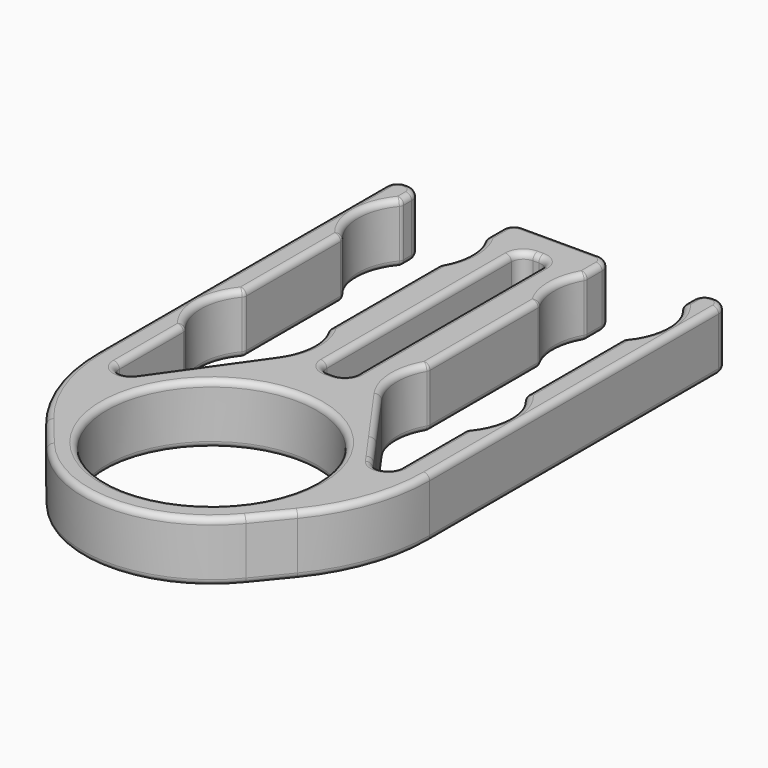
from build123d import *

# Parameters (mm, degrees)
F0_R         = 8.75
F0_W         = 2.5
F0_H         = 21.2536069062
F1_DEPTH     = 5
F2_R         = 1
F3_R         = 0.49999
F4_T1_DEPTH  = 5
F4_T4_ANGLE  = 39.3414951805
F4_T6_ANGLE  = 39.3414951805
F4_T8_ANGLE  = 39.3414951805
F4_T10_ANGLE = 39.3414951805


# Not quite as in the source:
# - a fillet or chamfer that OpenCascade refuses, or shapes differently, is made with other operations: its cross-section is extruded or revolved along the edge and cut away or added
# - a fillet or chamfer is up to 0.001 mm smaller than in the source, because OpenCascade refuses the exact size


with BuildPart() as f1:
    # F0 (on Top) → F1 (new body)
    with BuildSketch(Plane.XY):
        with BuildLine():
            ThreePointArc((-3.525, -3.1087577905), (-4.7, 0), (-3.525, 3.1087577905))
            Line((-3.525, 3.1087577905), (-3.525, 13.2912422095))
            ThreePointArc((-3.525, 13.2912422095), (-4.7, 16.4), (-3.525, 19.5087577905))
            Line((-3.525, 19.5087577905), (-3.525, 21.5087577905))
            Line((-3.525, 21.5087577905), (-5.7, 21.5087577905))
            Line((-5.7, 21.5087577905), (-5.7, 0))
            Line((-5.7, 0), (-5.7, -15))
            Line((-5.7, -15), (-0.1138489209, -21.8148672857))
            ThreePointArc((-0.1138489209, -21.8148672857), (8.2, -25.75), (16.5138489209, -21.8148672857))
            Line((16.5138489209, -21.8148672857), (22.1, -15))
            Line((22.1, -15), (22.1, 0))
            Line((22.1, 0), (22.1, 21.5087577905))
            Line((22.1, 21.5087577905), (19.925, 21.5087577905))
            Line((19.925, 21.5087577905), (19.925, 19.5087577905))
            ThreePointArc((19.925, 19.5087577905), (21.1, 16.4), (19.925, 13.2912422095))
            Line((19.925, 13.2912422095), (19.925, 3.1087577905))
            ThreePointArc((19.925, 3.1087577905), (21.1, 0), (19.925, -3.1087577905))
            Line((19.925, -3.1087577905), (19.925, -13.1087577905))
            Line((19.925, -13.1087577905), (17.6966700997, -9.9625644404))
            Line((17.6966700997, -9.9625644404), (16.1036863409, -7.713420403))
            Line((16.1036863409, -7.713420403), (12.5645563007, -2.7164998857))
            ThreePointArc((12.5645563007, -2.7164998857), (11.703188731, -0.1731008479), (12.375, 2.4268034531))
            Line((12.375, 2.4268034531), (12.375, 13.9731965469))
            ThreePointArc((12.375, 13.9731965469), (11.7, 16.4), (12.375, 18.8268034531))
            Line((12.375, 18.8268034531), (12.375, 21.5087577905))
            Line((12.375, 21.5087577905), (8.2, 21.5087577905))
            Line((8.2, 21.5087577905), (4.025, 21.5087577905))
            Line((4.025, 21.5087577905), (4.025, 18.8268034531))
            ThreePointArc((4.025, 18.8268034531), (4.7, 16.4), (4.025, 13.9731965469))
            Line((4.025, 13.9731965469), (4.025, 2.4268034531))
            ThreePointArc((4.025, 2.4268034531), (4.696811269, -0.1731008479), (3.8354436993, -2.7164998857))
            Line((3.8354436993, -2.7164998857), (0.2963136591, -7.713420403))
            Line((0.2963136591, -7.713420403), (-1.2966700997, -9.9625644404))
            Line((-1.2966700997, -9.9625644404), (-3.525, -13.1087577905))
            Line((-3.525, -13.1087577905), (-3.525, -3.1087577905))
        make_face()
        with Locations((8.2, -15)):
            Circle(F0_R, mode=Mode.SUBTRACT)
        with Locations((8.2, 8.2)):
            Rectangle(F0_W, F0_H, mode=Mode.SUBTRACT)
    extrude(amount=F1_DEPTH)

    # F2
    f2_edges = [f1.edges().sort_by_distance(p)[0] for p in [
        (-3.525, -13.108758, 2.5),
        (19.925, -13.108758, 2.5),
        (4.025, 21.508758, 2.5),
        (-5.7, 21.508758, 2.5),
        (-3.525, 21.508758, 2.5),
        (12.375, 21.508758, 2.5),
        (19.925, 21.508758, 2.5),
        (22.1, 21.508758, 2.5),
        (6.95, -2.426803, 2.5),
        (9.45, -2.426803, 2.5),
        (9.45, 18.826803, 2.5),
        (6.95, 18.826803, 2.5),
    ]]
    fillet(f2_edges, radius=F2_R)

    # F3 (radius 0.5 in the source; OpenCascade refuses exactly that, so slightly less here)
    f3_edges = [f1.edges().sort_by_distance(p)[0] for p in [
        (4.025, 19.667781, 5),
        (4.317893, 21.215865, 5),
        (4.7, 16.4, 5),
        (8.2, 21.508758, 5),
        (4.025, 8.2, 5),
        (12.082107, 21.215865, 5),
        (4.696811, -0.173101, 5),
        (12.375, 19.667781, 5),
        (1.063248, -6.630581, 5),
        (11.7, 16.4, 5),
        (-2.828272, -10.919588, 5),
        (12.375, 8.2, 5),
        (-3.525, -6.537721, 5),
        (11.703189, -0.173101, 5),
        (-4.7, 0, 5),
        (15.336752, -6.630581, 5),
        (-3.525, 8.2, 5),
        (19.228272, -10.919588, 5),
        (-4.7, 16.4, 5),
        (19.925, -6.537721, 5),
        (-3.525, 20.008758, 5),
        (21.1, 0, 5),
        (-3.817893, 21.215865, 5),
        (19.925, 8.2, 5),
        (-4.6125, 21.508758, 5),
        (21.1, 16.4, 5),
        (-5.407107, 21.215865, 5),
        (19.925, 20.008758, 5),
        (-5.7, 2.754379, 5),
        (20.217893, 21.215865, 5),
        (-2.906924, -18.407434, 5),
        (21.0125, 21.508758, 5),
        (8.2, -25.75, 5),
        (21.807107, 21.215865, 5),
        (19.306924, -18.407434, 5),
        (22.1, 2.754379, 5),
        (-0.55, -15, 5),
        (8.2, 18.826803, 5),
        (7.242893, 18.53391, 5),
        (9.157107, 18.53391, 5),
        (6.95, 8.2, 5),
        (9.45, 8.2, 5),
        (7.242893, -2.13391, 5),
        (9.157107, -2.13391, 5),
        (8.2, -2.426803, 5),
        (4.025, 19.667781, 0),
        (4.317893, 21.215865, 0),
        (4.7, 16.4, 0),
        (8.2, 21.508758, 0),
        (4.025, 8.2, 0),
        (12.082107, 21.215865, 0),
        (4.696811, -0.173101, 0),
        (12.375, 19.667781, 0),
        (1.063248, -6.630581, 0),
        (11.7, 16.4, 0),
        (-2.828272, -10.919588, 0),
        (12.375, 8.2, 0),
        (-3.525, -6.537721, 0),
        (11.703189, -0.173101, 0),
        (-4.7, 0, 0),
        (15.336752, -6.630581, 0),
        (-3.525, 8.2, 0),
        (19.228272, -10.919588, 0),
        (-4.7, 16.4, 0),
        (19.925, -6.537721, 0),
        (-3.525, 20.008758, 0),
        (21.1, 0, 0),
        (-3.817893, 21.215865, 0),
        (19.925, 8.2, 0),
        (-4.6125, 21.508758, 0),
        (21.1, 16.4, 0),
        (-5.407107, 21.215865, 0),
        (19.925, 20.008758, 0),
        (-5.7, 2.754379, 0),
        (20.217893, 21.215865, 0),
        (-2.906924, -18.407434, 0),
        (21.0125, 21.508758, 0),
        (8.2, -25.75, 0),
        (21.807107, 21.215865, 0),
        (19.306924, -18.407434, 0),
        (22.1, 2.754379, 0),
        (-0.55, -15, 0),
        (8.2, 18.826803, 0),
        (7.242893, 18.53391, 0),
        (9.157107, 18.53391, 0),
        (6.95, 8.2, 0),
        (9.45, 8.2, 0),
        (7.242893, -2.13391, 0),
        (9.157107, -2.13391, 0),
        (8.2, -2.426803, 0),
        (-3.525, 3.108758, 2.5),
        (-3.525, -3.108758, 2.5),
        (-3.525, 13.291242, 2.5),
        (-3.525, 19.508758, 2.5),
        (12.375, 13.973197, 2.5),
        (12.375, 18.826803, 2.5),
        (12.375, 2.426803, 2.5),
        (4.025, 2.426803, 2.5),
        (4.025, 13.973197, 2.5),
        (4.025, 18.826803, 2.5),
        (19.925, 19.508758, 2.5),
        (19.925, 13.291242, 2.5),
        (19.925, -3.108758, 2.5),
        (19.925, 3.108758, 2.5),
    ]]
    fillet(f3_edges, radius=F3_R)

    # F4: fillet of radius 15 on 2 edges, made by hand

    # F4_s2 → F4_t1 (cut)
    with BuildSketch(Plane.XY):
        with BuildLine():
            ThreePointArc((22.1, -9.6378609215), (21.2246378957, -14.6870791102), (18.7007194245, -19.1469780643))
            Line((18.7007194245, -19.1469780643), (22.1, -15))
            Line((22.1, -15), (22.1, -9.6378609215))
        make_face()
        with BuildLine():
            ThreePointArc((-2.3007194245, -19.1469780643), (-4.8246378957, -14.6870791102), (-5.7, -9.6378609215))
            Line((-5.7, -9.6378609215), (-5.7, -15))
            Line((-5.7, -15), (-2.3007194245, -19.1469780643))
        make_face()
    extrude(amount=F4_T1_DEPTH, mode=Mode.SUBTRACT)

    # F4_s3 → F4_t4 (revolve, cut)
    with BuildSketch(Plane(origin=(8.4627300816, -10.32417161, 0), x_dir=(0, 0, 1), z_dir=(0.6339411429, -0.773381295, 0))):
        with BuildLine():
            ThreePointArc((0, 13.4174005241), (0.1464436805, 13.7709468436), (0.49999, 13.9173905241))
            Line((0.49999, 13.9173905241), (0, 13.9173905241))
            Line((0, 13.9173905241), (0, 13.4174005241))
        make_face()
    revolve(axis=Axis((9.3, -9.6378609215, 0), (0, 0, -1)), revolution_arc=F4_T4_ANGLE, mode=Mode.SUBTRACT)

    # F4_s5 → F4_t6 (revolve, cut)
    with BuildSketch(Plane.XZ.offset(9.6378609215)):
        with BuildLine():
            ThreePointArc((-5.20001, 5), (-5.5535563195, 4.8535563195), (-5.7, 4.50001))
            Line((-5.7, 4.50001), (-5.7, 5))
            Line((-5.7, 5), (-5.20001, 5))
        make_face()
    revolve(axis=Axis((9.3, -9.6378609215, 5), (0, 0, 1)), revolution_arc=F4_T6_ANGLE, mode=Mode.SUBTRACT)

    # F4_s7 → F4_t8 (revolve, cut)
    with BuildSketch(Plane.XZ.offset(9.6378609215)):
        with BuildLine():
            ThreePointArc((21.60001, 0), (21.9535563195, 0.1464436805), (22.1, 0.49999))
            Line((22.1, 0.49999), (22.1, 0))
            Line((22.1, 0), (21.60001, 0))
        make_face()
    revolve(axis=Axis((7.1, -9.6378609215, 0), (0, 0, -1)), revolution_arc=F4_T8_ANGLE, mode=Mode.SUBTRACT)

    # F4_s9 → F4_t10 (revolve, cut)
    with BuildSketch(Plane(origin=(-1.8718755709, -2.2836087693, 0), x_dir=(0, 0, 1), z_dir=(-0.6339411429, -0.773381295, 0))):
        with BuildLine():
            ThreePointArc((5, -26.1008537615), (4.8535563195, -26.454400081), (4.50001, -26.6008437615))
            Line((4.50001, -26.6008437615), (5, -26.6008437615))
            Line((5, -26.6008437615), (5, -26.1008537615))
        make_face()
    revolve(axis=Axis((7.1, -9.6378609215, 5), (0, 0, 1)), revolution_arc=F4_T10_ANGLE, mode=Mode.SUBTRACT)


solid = f1.part
